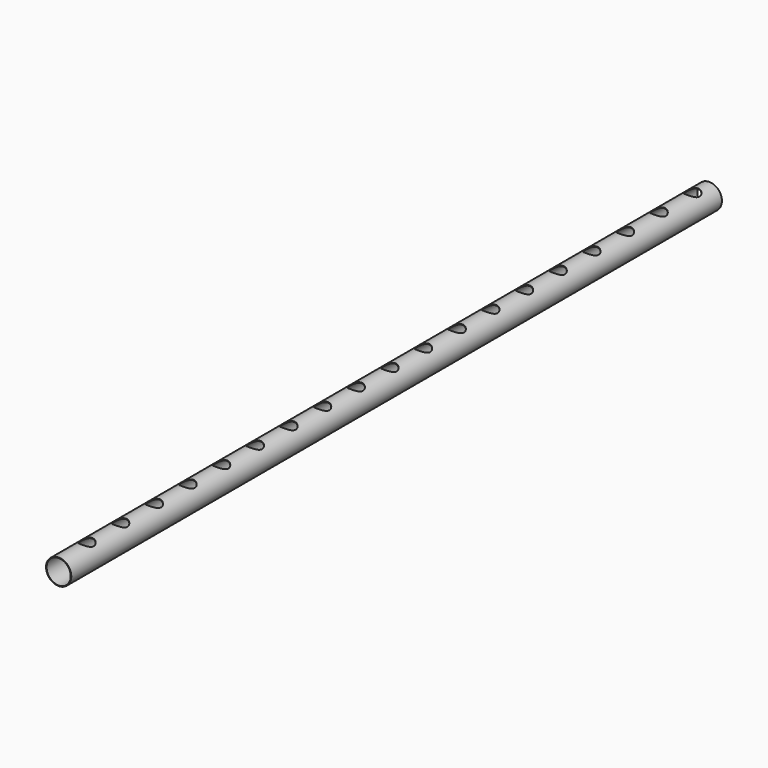
from build123d import *

# Parameters (mm, degrees)
F0_R     = 45
F0_R_2   = 43
F1_DEPTH = 1450
F4_D     = 50
F4_DEPTH = 50
F4_TIP   = 15.0215154757
F6_D     = 0.5
F6_DEPTH = 50
F6_TIP   = 0.1502151548


# Not quite as in the source:
# - a feature names something its author has since deleted; it is built from what else it names


with BuildPart() as f1:
    # F0 (on Front) → F1 (new body, symmetric)
    with BuildSketch(Plane.XZ):
        Circle(F0_R)
        Circle(F0_R_2, mode=Mode.SUBTRACT)
    extrude(amount=F1_DEPTH, both=True)

    # F4
    with Locations(Plane.XY.offset(45)):
        with Locations((0, -1325), (0, -1175), (0, -1025), (0, -875), (0, -725), (0, -575), (0, -425), (0, -275), (0, -125), (0, 25), (0, 175), (0, 325), (0, 475), (0, 625), (0, 775), (0, 925), (0, 1075), (0, 1225), (0, 1375)):
            Hole(F4_D / 2, depth=F4_DEPTH)
            with Locations((0, 0, -(F4_DEPTH + F4_TIP / 2))):  # 118° drill point
                Cone(0, F4_D / 2, F4_TIP, mode=Mode.SUBTRACT)

    # F6 (one way)
    with BuildSketch(Plane.XY):
        with Locations((0, 0)):
            Circle(F6_D / 2)
    extrude(amount=-F6_DEPTH, mode=Mode.SUBTRACT)
    with Locations(Plane.XY):
        with Locations((0, 0)):
            with Locations((0, 0, -(F6_DEPTH + F6_TIP / 2))):  # 118° drill point
                Cone(0, F6_D / 2, F6_TIP, mode=Mode.SUBTRACT)


solid = f1.part
